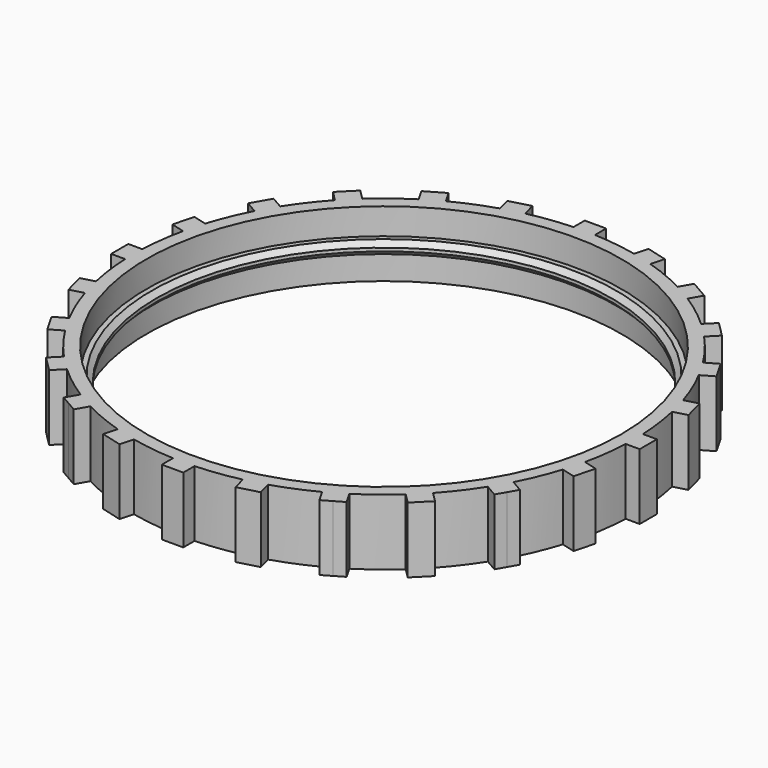
from build123d import *

# Parameters (mm, degrees)
F0_R     = 18.288
F1_DEPTH = 2.54
F0_R_2   = 17.526
F2_DEPTH = 0.508
F3_SIZE  = 0.381
F4_DEPTH = 2.54


# Not quite as in the source:
# - a feature names something its author has since deleted; it is built from what else it names


with BuildPart() as f1:
    # F0 (on Top) → F1 (new body, symmetric)
    with BuildSketch(Plane.XY):
        with BuildLine():
            ThreePointArc((19.2862771176, -0.8270011749), (19.2995687708, -0.4135955282), (19.304, 0))
            ThreePointArc((19.304, 0), (19.2995687708, 0.4135955282), (19.2862771176, 0.8270011749))
            ThreePointArc((19.2862771176, 0.8270011749), (19.138851604, 2.5196776146), (18.8431568152, 4.1928340339))
            ThreePointArc((18.8431568152, 4.1928340339), (18.6462321507, 4.9962428467), (18.4150695065, 5.7904776204))
            ThreePointArc((18.4150695065, 5.7904776204), (17.8345704956, 7.3873209784), (17.1159065157, 8.9269345324))
            ThreePointArc((17.1159065157, 8.9269345324), (16.7177543947, 9.652), (16.2889053408, 10.3593425852))
            ThreePointArc((16.2889053408, 10.3593425852), (15.314892881, 11.7515306256), (14.2222354725, 13.0526791949))
            ThreePointArc((14.2222354725, 13.0526791949), (13.649989304, 13.649989304), (13.0526791949, 14.2222354725))
            ThreePointArc((13.0526791949, 14.2222354725), (11.7515306256, 15.314892881), (10.3593425852, 16.2889053408))
            ThreePointArc((10.3593425852, 16.2889053408), (9.652, 16.7177543947), (8.9269345324, 17.1159065157))
            ThreePointArc((8.9269345324, 17.1159065157), (7.3873209784, 17.8345704956), (5.7904776204, 18.4150695065))
            ThreePointArc((5.7904776204, 18.4150695065), (4.9962428467, 18.6462321507), (4.1928340339, 18.8431568152))
            ThreePointArc((4.1928340339, 18.8431568152), (2.5196776146, 19.138851604), (0.8270011749, 19.2862771176))
            ThreePointArc((0.8270011749, 19.2862771176), (0, 19.304), (-0.8270011749, 19.2862771176))
            ThreePointArc((-0.8270011749, 19.2862771176), (-2.5196776146, 19.138851604), (-4.1928340339, 18.8431568152))
            ThreePointArc((-4.1928340339, 18.8431568152), (-4.9962428467, 18.6462321507), (-5.7904776204, 18.4150695065))
            ThreePointArc((-5.7904776204, 18.4150695065), (-7.3873209784, 17.8345704956), (-8.9269345324, 17.1159065157))
            ThreePointArc((-8.9269345324, 17.1159065157), (-9.652, 16.7177543947), (-10.3593425852, 16.2889053408))
            ThreePointArc((-10.3593425852, 16.2889053408), (-11.7515306256, 15.314892881), (-13.0526791949, 14.2222354725))
            ThreePointArc((-13.0526791949, 14.2222354725), (-13.649989304, 13.649989304), (-14.2222354725, 13.0526791949))
            ThreePointArc((-14.2222354725, 13.0526791949), (-15.314892881, 11.7515306256), (-16.2889053408, 10.3593425852))
            ThreePointArc((-16.2889053408, 10.3593425852), (-16.7177543947, 9.652), (-17.1159065157, 8.9269345324))
            ThreePointArc((-17.1159065157, 8.9269345324), (-17.8345704956, 7.3873209784), (-18.4150695065, 5.7904776204))
            ThreePointArc((-18.4150695065, 5.7904776204), (-18.6462321507, 4.9962428467), (-18.8431568152, 4.1928340339))
            ThreePointArc((-18.8431568152, 4.1928340339), (-19.138851604, 2.5196776146), (-19.2862771176, 0.8270011749))
            ThreePointArc((-19.2862771176, 0.8270011749), (-19.304, 0), (-19.2862771176, -0.8270011749))
            ThreePointArc((-19.2862771176, -0.8270011749), (-19.138851604, -2.5196776146), (-18.8431568152, -4.1928340339))
            ThreePointArc((-18.8431568152, -4.1928340339), (-18.6462321507, -4.9962428467), (-18.4150695065, -5.7904776204))
            ThreePointArc((-18.4150695065, -5.7904776204), (-17.8345704956, -7.3873209784), (-17.1159065157, -8.9269345324))
            ThreePointArc((-17.1159065157, -8.9269345324), (-16.7177543947, -9.652), (-16.2889053408, -10.3593425852))
            ThreePointArc((-16.2889053408, -10.3593425852), (-15.314892881, -11.7515306256), (-14.2222354725, -13.0526791949))
            ThreePointArc((-14.2222354725, -13.0526791949), (-13.649989304, -13.649989304), (-13.0526791949, -14.2222354725))
            ThreePointArc((-13.0526791949, -14.2222354725), (-11.7515306256, -15.314892881), (-10.3593425852, -16.2889053408))
            ThreePointArc((-10.3593425852, -16.2889053408), (-9.652, -16.7177543947), (-8.9269345324, -17.1159065157))
            ThreePointArc((-8.9269345324, -17.1159065157), (-7.3873209784, -17.8345704956), (-5.7904776204, -18.4150695065))
            ThreePointArc((-5.7904776204, -18.4150695065), (-4.9962428467, -18.6462321507), (-4.1928340339, -18.8431568152))
            ThreePointArc((-4.1928340339, -18.8431568152), (-2.5196776146, -19.138851604), (-0.8270011749, -19.2862771176))
            ThreePointArc((-0.8270011749, -19.2862771176), (0, -19.304), (0.8270011749, -19.2862771176))
            ThreePointArc((0.8270011749, -19.2862771176), (2.5196776146, -19.138851604), (4.1928340339, -18.8431568152))
            ThreePointArc((4.1928340339, -18.8431568152), (4.9962428467, -18.6462321507), (5.7904776204, -18.4150695065))
            ThreePointArc((5.7904776204, -18.4150695065), (7.3873209784, -17.8345704956), (8.9269345324, -17.1159065157))
            ThreePointArc((8.9269345324, -17.1159065157), (9.652, -16.7177543947), (10.3593425852, -16.2889053408))
            ThreePointArc((10.3593425852, -16.2889053408), (11.7515306256, -15.314892881), (13.0526791949, -14.2222354725))
            ThreePointArc((13.0526791949, -14.2222354725), (13.649989304, -13.649989304), (14.2222354725, -13.0526791949))
            ThreePointArc((14.2222354725, -13.0526791949), (15.314892881, -11.7515306256), (16.2889053408, -10.3593425852))
            ThreePointArc((16.2889053408, -10.3593425852), (16.7177543947, -9.652), (17.1159065157, -8.9269345324))
            ThreePointArc((17.1159065157, -8.9269345324), (17.8345704956, -7.3873209784), (18.4150695065, -5.7904776204))
            ThreePointArc((18.4150695065, -5.7904776204), (18.6462321507, -4.9962428467), (18.8431568152, -4.1928340339))
            ThreePointArc((18.8431568152, -4.1928340339), (19.138851604, -2.5196776146), (19.2862771176, -0.8270011749))
        make_face()
        Circle(F0_R, mode=Mode.SUBTRACT)
        with BuildLine():
            ThreePointArc((19.2862771176, 0.8270011749), (19.2995687708, 0.4135955282), (19.304, 0))
            ThreePointArc((19.304, 0), (19.2995687708, -0.4135955282), (19.2862771176, -0.8270011749))
            Line((19.2862771176, -0.8270011749), (20.3670533557, -0.8270011749))
            Line((20.3670533557, -0.8270011749), (20.3670533557, 0))
            Line((20.3670533557, 0), (20.3670533557, 0.8270011749))
            Line((20.3670533557, 0.8270011749), (19.2862771176, 0.8270011749))
        make_face()
        with BuildLine():
            ThreePointArc((18.4150695065, 5.7904776204), (18.6462321507, 4.9962428467), (18.8431568152, 4.1928340339))
            Line((18.8431568152, 4.1928340339), (19.8871064961, 4.4725595079))
            Line((19.8871064961, 4.4725595079), (19.6730628417, 5.2713813011))
            Line((19.6730628417, 5.2713813011), (19.4590191873, 6.0702030943))
            Line((19.4590191873, 6.0702030943), (18.4150695065, 5.7904776204))
        make_face()
        with BuildLine():
            Line((19.8871064961, -4.4725595079), (18.8431568152, -4.1928340339))
            ThreePointArc((18.8431568152, -4.1928340339), (18.6462321507, -4.9962428467), (18.4150695065, -5.7904776204))
            Line((18.4150695065, -5.7904776204), (19.4590191873, -6.0702030943))
            Line((19.4590191873, -6.0702030943), (19.6730628417, -5.2713813011))
            Line((19.6730628417, -5.2713813011), (19.8871064961, -4.4725595079))
        make_face()
        with BuildLine():
            ThreePointArc((16.2889053408, 10.3593425852), (16.7177543947, 9.652), (17.1159065157, 8.9269345324))
            Line((17.1159065157, 8.9269345324), (18.0518861937, 9.4673226514))
            Line((18.0518861937, 9.4673226514), (17.6383856063, 10.1835266779))
            Line((17.6383856063, 10.1835266779), (17.2248850188, 10.8997307043))
            Line((17.2248850188, 10.8997307043), (16.2889053408, 10.3593425852))
        make_face()
        with BuildLine():
            Line((18.0518861937, -9.4673226514), (17.1159065157, -8.9269345324))
            ThreePointArc((17.1159065157, -8.9269345324), (16.7177543947, -9.652), (16.2889053408, -10.3593425852))
            Line((16.2889053408, -10.3593425852), (17.2248850188, -10.8997307043))
            Line((17.2248850188, -10.8997307043), (17.6383856063, -10.1835266779))
            Line((17.6383856063, -10.1835266779), (18.0518861937, -9.4673226514))
        make_face()
        with BuildLine():
            ThreePointArc((13.0526791949, 14.2222354725), (13.649989304, 13.649989304), (14.2222354725, 13.0526791949))
            Line((14.2222354725, 13.0526791949), (14.9864596794, 13.8169034018))
            Line((14.9864596794, 13.8169034018), (14.4016815406, 14.4016815406))
            Line((14.4016815406, 14.4016815406), (13.8169034018, 14.9864596794))
            Line((13.8169034018, 14.9864596794), (13.0526791949, 14.2222354725))
        make_face()
        with BuildLine():
            Line((14.9864596794, -13.8169034018), (14.2222354725, -13.0526791949))
            ThreePointArc((14.2222354725, -13.0526791949), (13.649989304, -13.649989304), (13.0526791949, -14.2222354725))
            Line((13.0526791949, -14.2222354725), (13.8169034018, -14.9864596794))
            Line((13.8169034018, -14.9864596794), (14.4016815406, -14.4016815406))
            Line((14.4016815406, -14.4016815406), (14.9864596794, -13.8169034018))
        make_face()
        with BuildLine():
            ThreePointArc((8.9269345324, 17.1159065157), (9.652, 16.7177543947), (10.3593425852, 16.2889053408))
            Line((10.3593425852, 16.2889053408), (10.8997307043, 17.2248850188))
            Line((10.8997307043, 17.2248850188), (10.1835266779, 17.6383856063))
            Line((10.1835266779, 17.6383856063), (9.4673226514, 18.0518861937))
            Line((9.4673226514, 18.0518861937), (8.9269345324, 17.1159065157))
        make_face()
        with BuildLine():
            Line((10.8997307043, -17.2248850188), (10.3593425852, -16.2889053408))
            ThreePointArc((10.3593425852, -16.2889053408), (9.652, -16.7177543947), (8.9269345324, -17.1159065157))
            Line((8.9269345324, -17.1159065157), (9.4673226514, -18.0518861937))
            Line((9.4673226514, -18.0518861937), (10.1835266779, -17.6383856063))
            Line((10.1835266779, -17.6383856063), (10.8997307043, -17.2248850188))
        make_face()
        with BuildLine():
            ThreePointArc((4.1928340339, 18.8431568152), (4.9962428467, 18.6462321507), (5.7904776204, 18.4150695065))
            Line((5.7904776204, 18.4150695065), (6.0702030943, 19.4590191873))
            Line((6.0702030943, 19.4590191873), (5.2713813011, 19.6730628417))
            Line((5.2713813011, 19.6730628417), (4.4725595079, 19.8871064961))
            Line((4.4725595079, 19.8871064961), (4.1928340339, 18.8431568152))
        make_face()
        with BuildLine():
            Line((6.0702030943, -19.4590191873), (5.7904776204, -18.4150695065))
            ThreePointArc((5.7904776204, -18.4150695065), (4.9962428467, -18.6462321507), (4.1928340339, -18.8431568152))
            Line((4.1928340339, -18.8431568152), (4.4725595079, -19.8871064961))
            Line((4.4725595079, -19.8871064961), (5.2713813011, -19.6730628417))
            Line((5.2713813011, -19.6730628417), (6.0702030943, -19.4590191873))
        make_face()
        with BuildLine():
            ThreePointArc((-0.8270011749, 19.2862771176), (0, 19.304), (0.8270011749, 19.2862771176))
            Line((0.8270011749, 19.2862771176), (0.8270011749, 20.3670533557))
            Line((0.8270011749, 20.3670533557), (0, 20.3670533557))
            Line((0, 20.3670533557), (-0.8270011749, 20.3670533557))
            Line((-0.8270011749, 20.3670533557), (-0.8270011749, 19.2862771176))
        make_face()
        with BuildLine():
            Line((0.8270011749, -20.3670533557), (0.8270011749, -19.2862771176))
            ThreePointArc((0.8270011749, -19.2862771176), (0, -19.304), (-0.8270011749, -19.2862771176))
            Line((-0.8270011749, -19.2862771176), (-0.8270011749, -20.3670533557))
            Line((-0.8270011749, -20.3670533557), (0, -20.3670533557))
            Line((0, -20.3670533557), (0.8270011749, -20.3670533557))
        make_face()
        with BuildLine():
            ThreePointArc((-5.7904776204, 18.4150695065), (-4.9962428467, 18.6462321507), (-4.1928340339, 18.8431568152))
            Line((-4.1928340339, 18.8431568152), (-4.4725595079, 19.8871064961))
            Line((-4.4725595079, 19.8871064961), (-5.2713813011, 19.6730628417))
            Line((-5.2713813011, 19.6730628417), (-6.0702030943, 19.4590191873))
            Line((-6.0702030943, 19.4590191873), (-5.7904776204, 18.4150695065))
        make_face()
        with BuildLine():
            Line((-4.4725595079, -19.8871064961), (-4.1928340339, -18.8431568152))
            ThreePointArc((-4.1928340339, -18.8431568152), (-4.9962428467, -18.6462321507), (-5.7904776204, -18.4150695065))
            Line((-5.7904776204, -18.4150695065), (-6.0702030943, -19.4590191873))
            Line((-6.0702030943, -19.4590191873), (-5.2713813011, -19.6730628417))
            Line((-5.2713813011, -19.6730628417), (-4.4725595079, -19.8871064961))
        make_face()
        with BuildLine():
            ThreePointArc((-10.3593425852, 16.2889053408), (-9.652, 16.7177543947), (-8.9269345324, 17.1159065157))
            Line((-8.9269345324, 17.1159065157), (-9.4673226514, 18.0518861937))
            Line((-9.4673226514, 18.0518861937), (-10.1835266779, 17.6383856063))
            Line((-10.1835266779, 17.6383856063), (-10.8997307043, 17.2248850188))
            Line((-10.8997307043, 17.2248850188), (-10.3593425852, 16.2889053408))
        make_face()
        with BuildLine():
            Line((-9.4673226514, -18.0518861937), (-8.9269345324, -17.1159065157))
            ThreePointArc((-8.9269345324, -17.1159065157), (-9.652, -16.7177543947), (-10.3593425852, -16.2889053408))
            Line((-10.3593425852, -16.2889053408), (-10.8997307043, -17.2248850188))
            Line((-10.8997307043, -17.2248850188), (-10.1835266779, -17.6383856063))
            Line((-10.1835266779, -17.6383856063), (-9.4673226514, -18.0518861937))
        make_face()
        with BuildLine():
            ThreePointArc((-14.2222354725, 13.0526791949), (-13.649989304, 13.649989304), (-13.0526791949, 14.2222354725))
            Line((-13.0526791949, 14.2222354725), (-13.8169034018, 14.9864596794))
            Line((-13.8169034018, 14.9864596794), (-14.4016815406, 14.4016815406))
            Line((-14.4016815406, 14.4016815406), (-14.9864596794, 13.8169034018))
            Line((-14.9864596794, 13.8169034018), (-14.2222354725, 13.0526791949))
        make_face()
        with BuildLine():
            Line((-13.8169034018, -14.9864596794), (-13.0526791949, -14.2222354725))
            ThreePointArc((-13.0526791949, -14.2222354725), (-13.649989304, -13.649989304), (-14.2222354725, -13.0526791949))
            Line((-14.2222354725, -13.0526791949), (-14.9864596794, -13.8169034018))
            Line((-14.9864596794, -13.8169034018), (-14.4016815406, -14.4016815406))
            Line((-14.4016815406, -14.4016815406), (-13.8169034018, -14.9864596794))
        make_face()
        with BuildLine():
            ThreePointArc((-17.1159065157, 8.9269345324), (-16.7177543947, 9.652), (-16.2889053408, 10.3593425852))
            Line((-16.2889053408, 10.3593425852), (-17.2248850188, 10.8997307043))
            Line((-17.2248850188, 10.8997307043), (-17.6383856063, 10.1835266779))
            Line((-17.6383856063, 10.1835266779), (-18.0518861937, 9.4673226514))
            Line((-18.0518861937, 9.4673226514), (-17.1159065157, 8.9269345324))
        make_face()
        with BuildLine():
            Line((-17.2248850188, -10.8997307043), (-16.2889053408, -10.3593425852))
            ThreePointArc((-16.2889053408, -10.3593425852), (-16.7177543947, -9.652), (-17.1159065157, -8.9269345324))
            Line((-17.1159065157, -8.9269345324), (-18.0518861937, -9.4673226514))
            Line((-18.0518861937, -9.4673226514), (-17.6383856063, -10.1835266779))
            Line((-17.6383856063, -10.1835266779), (-17.2248850188, -10.8997307043))
        make_face()
        with BuildLine():
            ThreePointArc((-18.8431568152, 4.1928340339), (-18.6462321507, 4.9962428467), (-18.4150695065, 5.7904776204))
            Line((-18.4150695065, 5.7904776204), (-19.4590191873, 6.0702030943))
            Line((-19.4590191873, 6.0702030943), (-19.6730628417, 5.2713813011))
            Line((-19.6730628417, 5.2713813011), (-19.8871064961, 4.4725595079))
            Line((-19.8871064961, 4.4725595079), (-18.8431568152, 4.1928340339))
        make_face()
        with BuildLine():
            Line((-19.4590191873, -6.0702030943), (-18.4150695065, -5.7904776204))
            ThreePointArc((-18.4150695065, -5.7904776204), (-18.6462321507, -4.9962428467), (-18.8431568152, -4.1928340339))
            Line((-18.8431568152, -4.1928340339), (-19.8871064961, -4.4725595079))
            Line((-19.8871064961, -4.4725595079), (-19.6730628417, -5.2713813011))
            Line((-19.6730628417, -5.2713813011), (-19.4590191873, -6.0702030943))
        make_face()
        with BuildLine():
            ThreePointArc((-19.2862771176, -0.8270011749), (-19.304, 0), (-19.2862771176, 0.8270011749))
            Line((-19.2862771176, 0.8270011749), (-20.3670533557, 0.8270011749))
            Line((-20.3670533557, 0.8270011749), (-20.3670533557, 0))
            Line((-20.3670533557, 0), (-20.3670533557, -0.8270011749))
            Line((-20.3670533557, -0.8270011749), (-19.2862771176, -0.8270011749))
        make_face()
    extrude(amount=F1_DEPTH, both=True)

    # F0 (on Top) → F2 (join, symmetric)
    with BuildSketch(Plane.XY):
        Circle(F0_R)
        Circle(F0_R_2, mode=Mode.SUBTRACT)
    extrude(amount=F2_DEPTH, both=True)

    # F3
    f3_edges = [f1.edges().sort_by_distance(p)[0] for p in [
        (-17.526, 0, 0.508),
        (17.526, 0, 0),
        (-17.526, 0, -0.508),
    ]]
    chamfer(f3_edges, length=F3_SIZE)

    # F0 (on Top) → F4 (join, symmetric)
    with BuildSketch(Plane.XY):
        with BuildLine():
            ThreePointArc((8.9269345324, 17.1159065157), (9.652, 16.7177543947), (10.3593425852, 16.2889053408))
            Line((10.3593425852, 16.2889053408), (10.8997307043, 17.2248850188))
            Line((10.8997307043, 17.2248850188), (10.1835266779, 17.6383856063))
            Line((10.1835266779, 17.6383856063), (9.4673226514, 18.0518861937))
            Line((9.4673226514, 18.0518861937), (8.9269345324, 17.1159065157))
        make_face()
        with BuildLine():
            ThreePointArc((4.1928340339, 18.8431568152), (4.9962428467, 18.6462321507), (5.7904776204, 18.4150695065))
            Line((5.7904776204, 18.4150695065), (6.0702030943, 19.4590191873))
            Line((6.0702030943, 19.4590191873), (5.2713813011, 19.6730628417))
            Line((5.2713813011, 19.6730628417), (4.4725595079, 19.8871064961))
            Line((4.4725595079, 19.8871064961), (4.1928340339, 18.8431568152))
        make_face()
        with BuildLine():
            ThreePointArc((-0.8270011749, 19.2862771176), (0, 19.304), (0.8270011749, 19.2862771176))
            Line((0.8270011749, 19.2862771176), (0.8270011749, 20.3670533557))
            Line((0.8270011749, 20.3670533557), (0, 20.3670533557))
            Line((0, 20.3670533557), (-0.8270011749, 20.3670533557))
            Line((-0.8270011749, 20.3670533557), (-0.8270011749, 19.2862771176))
        make_face()
        with BuildLine():
            ThreePointArc((-5.7904776204, 18.4150695065), (-4.9962428467, 18.6462321507), (-4.1928340339, 18.8431568152))
            Line((-4.1928340339, 18.8431568152), (-4.4725595079, 19.8871064961))
            Line((-4.4725595079, 19.8871064961), (-5.2713813011, 19.6730628417))
            Line((-5.2713813011, 19.6730628417), (-6.0702030943, 19.4590191873))
            Line((-6.0702030943, 19.4590191873), (-5.7904776204, 18.4150695065))
        make_face()
        with BuildLine():
            ThreePointArc((-10.3593425852, 16.2889053408), (-9.652, 16.7177543947), (-8.9269345324, 17.1159065157))
            Line((-8.9269345324, 17.1159065157), (-9.4673226514, 18.0518861937))
            Line((-9.4673226514, 18.0518861937), (-10.1835266779, 17.6383856063))
            Line((-10.1835266779, 17.6383856063), (-10.8997307043, 17.2248850188))
            Line((-10.8997307043, 17.2248850188), (-10.3593425852, 16.2889053408))
        make_face()
        with BuildLine():
            ThreePointArc((-14.2222354725, 13.0526791949), (-13.649989304, 13.649989304), (-13.0526791949, 14.2222354725))
            Line((-13.0526791949, 14.2222354725), (-13.8169034018, 14.9864596794))
            Line((-13.8169034018, 14.9864596794), (-14.4016815406, 14.4016815406))
            Line((-14.4016815406, 14.4016815406), (-14.9864596794, 13.8169034018))
            Line((-14.9864596794, 13.8169034018), (-14.2222354725, 13.0526791949))
        make_face()
        with BuildLine():
            ThreePointArc((-17.1159065157, 8.9269345324), (-16.7177543947, 9.652), (-16.2889053408, 10.3593425852))
            Line((-16.2889053408, 10.3593425852), (-17.2248850188, 10.8997307043))
            Line((-17.2248850188, 10.8997307043), (-17.6383856063, 10.1835266779))
            Line((-17.6383856063, 10.1835266779), (-18.0518861937, 9.4673226514))
            Line((-18.0518861937, 9.4673226514), (-17.1159065157, 8.9269345324))
        make_face()
        with BuildLine():
            ThreePointArc((-18.8431568152, 4.1928340339), (-18.6462321507, 4.9962428467), (-18.4150695065, 5.7904776204))
            Line((-18.4150695065, 5.7904776204), (-19.4590191873, 6.0702030943))
            Line((-19.4590191873, 6.0702030943), (-19.6730628417, 5.2713813011))
            Line((-19.6730628417, 5.2713813011), (-19.8871064961, 4.4725595079))
            Line((-19.8871064961, 4.4725595079), (-18.8431568152, 4.1928340339))
        make_face()
    extrude(amount=F4_DEPTH, both=True)


solid = f1.part
